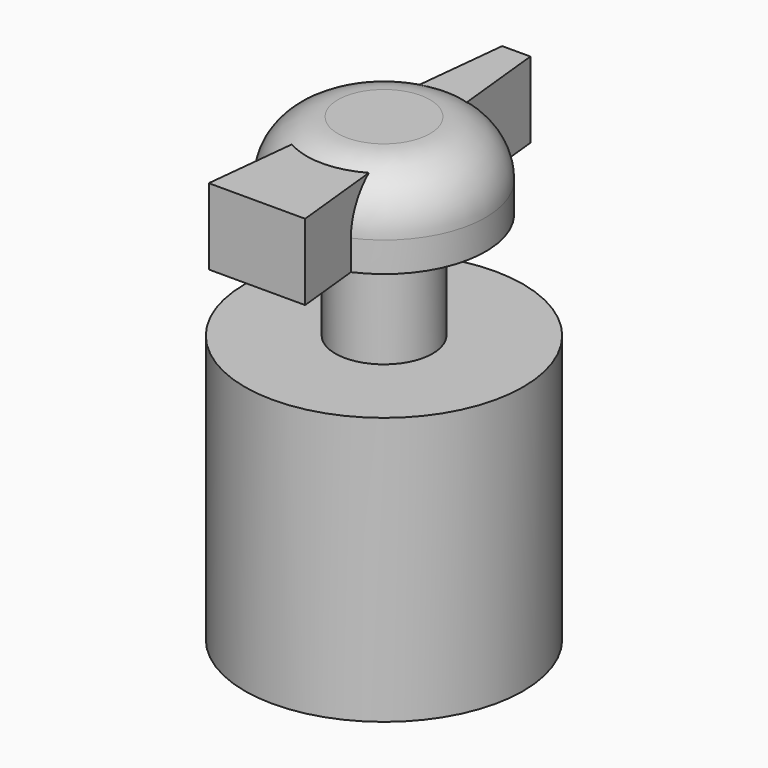
from build123d import *

# Parameters (mm, degrees)
F0_R     = 9.5
F1_DEPTH = 8
F2_R     = 5.2
F4_DEPTH = 7.1
F5_R     = 4.55
F6_DEPTH = 35
F7_R     = 13
F7_R_2   = 4.55
F8_DEPTH = 25


with BuildPart() as f1:
    # F0 (on Top) → F1 (new body)
    with BuildSketch(Plane.XY):
        Circle(F0_R)
    extrude(amount=F1_DEPTH)

    # F2
    f2_edges = [f1.edges().sort_by_distance(p)[0] for p in [
        (-9.5, 0, 8),
    ]]
    fillet(f2_edges, radius=F2_R)

    # F3 (on Top) → F4 (join)
    with BuildSketch(Plane.XY):
        Polygon((4.5, -14.8323969742), (1.3178354695, 15.4438761221), (-1.3178354695, 15.4438761221), (-4.5, -14.8323969742), align=None)
    extrude(amount=F4_DEPTH)

    # F5 (on face) → F6 (join)
    with BuildSketch(Plane(origin=(0, 0, 0), x_dir=(1, 0, 0), z_dir=(0, 0, -1))):
        Circle(F5_R)
    extrude(amount=F6_DEPTH)

    # F7 (on face) → F8 (join)
    with BuildSketch(Plane(origin=(0, 0, -35), x_dir=(1, 0, 0), z_dir=(0, 0, -1))):
        Circle(F7_R)
        Circle(F7_R_2, mode=Mode.SUBTRACT)
    extrude(amount=-F8_DEPTH)


solid = f1.part
